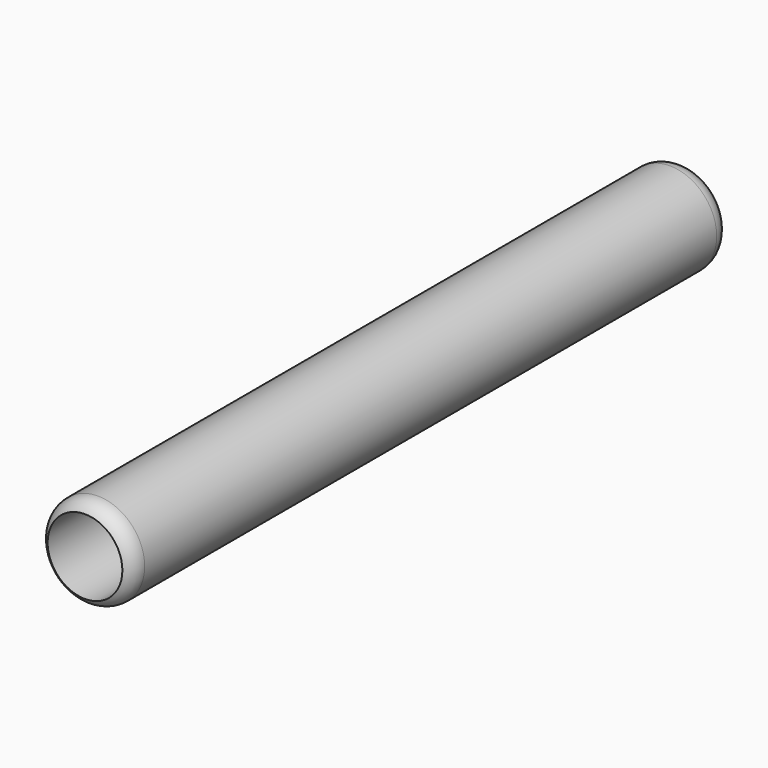
from build123d import *

# Parameters (mm, degrees)
F0_R     = 1.25
F0_R_2   = 1
F1_DEPTH = 20


# Not quite as in the source:
# - a fillet or chamfer that OpenCascade refuses, or shapes differently, is made with other operations: its cross-section is extruded or revolved along the edge and cut away or added


with BuildPart() as f1:
    # F0 (on Front) → F1 (new body)
    with BuildSketch(Plane.XZ):
        with Locations((-30.6629948318, 34.7370989621)):
            Circle(F0_R)
        with Locations((-30.6629948318, 34.7370989621)):
            Circle(F0_R_2, mode=Mode.SUBTRACT)
    extrude(amount=F1_DEPTH)

    # F2: fillet of radius 0.5 on 1 edges, made by hand

    # F2_s1 → F2_t2 (revolve, cut)
    with BuildSketch(Plane.XY.offset(34.7370989621)):
        with BuildLine():
            ThreePointArc((-29.4129948318, -19.5669872981), (-29.4799821299, -19.8169872981), (-29.6629948318, -20))
            Line((-29.6629948318, -20), (-29.4129948318, -20))
            Line((-29.4129948318, -20), (-29.4129948318, -19.5669872981))
        make_face()
    revolve(axis=Axis((-30.6629948318, -20, 34.7370989621), (0, -1, 0)), mode=Mode.SUBTRACT)

    # F3: fillet of radius 0.5 on 1 edges, made by hand

    # F3_s1 → F3_t2 (revolve, cut)
    with BuildSketch(Plane.XY.offset(34.7370989621)):
        with BuildLine():
            ThreePointArc((-29.4129948318, -0.4330127019), (-29.4799821299, -0.1830127019), (-29.6629948318, 0))
            Line((-29.6629948318, 0), (-29.4129948318, 0))
            Line((-29.4129948318, 0), (-29.4129948318, -0.4330127019))
        make_face()
    revolve(axis=Axis((-30.6629948318, 0, 34.7370989621), (0, -1, 0)), mode=Mode.SUBTRACT)


solid = f1.part
